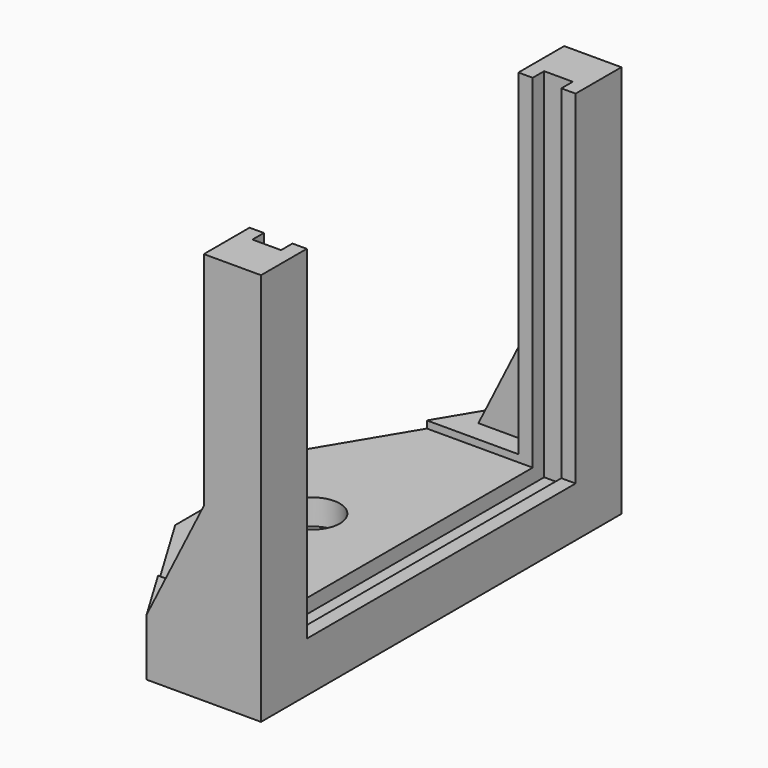
from build123d import *

# Parameters (mm, degrees)
F0_W           = 20
F0_H           = 63
F1_DEPTH       = 8
F2_W           = 63
F2_H           = 55
F3_DEPTH       = 8
F5_D           = 4.572
F5_CBORE_D     = 7.62
F5_CBORE_DEPTH = 4.572
F6_W           = 47
F6_H           = 48
F7_DEPTH       = 28.001
F9_W           = 4
F9_H           = 51
F10_DEPTH      = 50
F12_DEPTH      = 5
F14_DEPTH      = 5
F16_DEPTH      = 25


# Not quite as in the source:
# - a feature names something its author has since deleted; it is built from what else it names


with BuildPart() as f1:
    # F0 (on Top) → F1 (new body)
    with BuildSketch(Plane.XY):
        Rectangle(F0_W, F0_H)
    extrude(amount=F1_DEPTH)

    # F2 (on face) → F3 (join)
    with BuildSketch(Plane.YZ.offset(10)):
        with Locations((0, 27.5)):
            Rectangle(F2_W, F2_H)
    extrude(amount=F3_DEPTH)

    # F5 (through all)
    with Locations(Plane.XY.offset(8)):
        with Locations((0, 0)):
            CounterBoreHole(F5_D / 2, F5_CBORE_D / 2, F5_CBORE_DEPTH)

    # F6 (on face) → F7 (cut, through all)
    with BuildSketch(Plane.YZ.offset(18)):
        with Locations((0, 31)):
            Rectangle(F6_W, F6_H)
    extrude(amount=-F7_DEPTH, mode=Mode.SUBTRACT)

    # F9 (on 3pt) → F10 (cut)
    with BuildSketch(Plane(origin=(0, 0, 55), x_dir=(1, 0, 0), z_dir=(0, 0, -1))):
        with Locations((14, 0)):
            Rectangle(F9_W, F9_H)
    extrude(amount=F10_DEPTH, mode=Mode.SUBTRACT)

    # F11 (on face) → F12 (join)
    with BuildSketch(Plane.XZ.offset(31.5)):
        Polygon((2, 8), (10, 8), (10, 24), align=None)
    extrude(amount=-F12_DEPTH)

    # F13 (on face) → F14 (join)
    with BuildSketch(Plane(origin=(0, 31.5, 0), x_dir=(-1, 0, 0), z_dir=(0, 1, 0))):
        Polygon((-10, 24), (-10, 8), (-2, 8), align=None)
    extrude(amount=-F14_DEPTH)

    # F15 (on face) → F16 (cut)
    with BuildSketch(Plane.XY.offset(8)):
        Polygon((-10, 11.5), (2, 31.5), (-10, 31.5), align=None)
        Polygon((-10, -11.5), (-10, -31.5), (2, -31.5), align=None)
    extrude(amount=-F16_DEPTH, mode=Mode.SUBTRACT)


solid = f1.part
